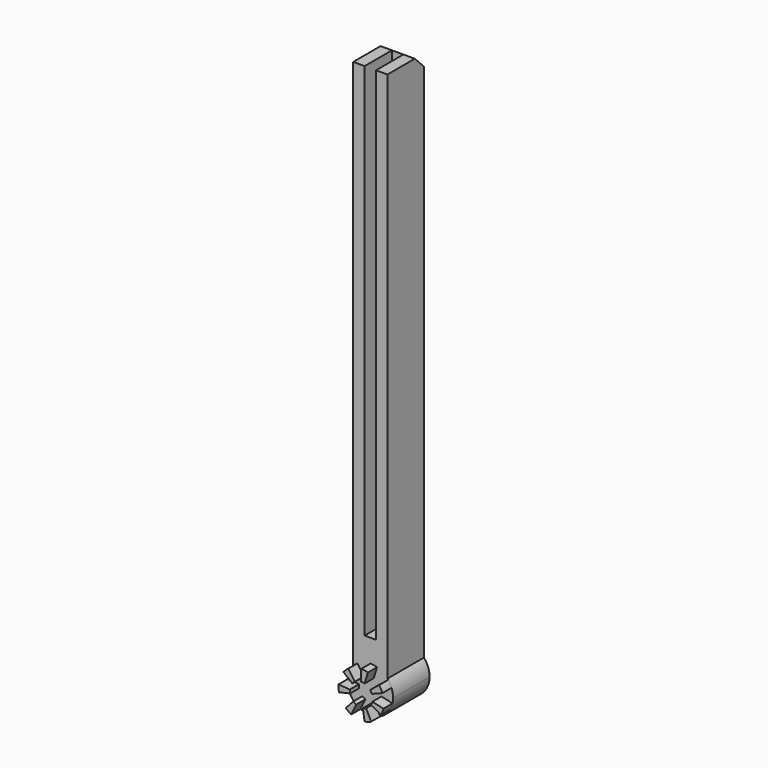
from build123d import *

# Parameters (mm, degrees)
F1_DEPTH = 12.7
F2_W     = 3.175
F2_H     = 9.525
F3_DEPTH = 139.7
F5_DEPTH = 3.175
F6_R     = 3.96875
F7_DEPTH = 3.175
F8_SIZE  = 3.17499


# Not quite as in the source:
# - a fillet or chamfer is up to 0.001 mm smaller than in the source, because OpenCascade refuses the exact size


with BuildPart() as f1:
    # F0 (on Front) → F1 (new body)
    with BuildSketch(Plane.XZ):
        with BuildLine():
            Line((0, 152.4), (0, 4.2001302063))
            ThreePointArc((0, 4.2001302063), (4.7625, 6.35), (9.525, 4.2001302063))
            Line((9.525, 4.2001302063), (9.525, 152.4))
            Line((9.525, 152.4), (0, 152.4))
        make_face()
        with BuildLine():
            Line((0, 4.2001302063), (0, 0))
            Line((0, 0), (9.525, 0))
            Line((9.525, 0), (9.525, 4.2001302063))
            ThreePointArc((9.525, 4.2001302063), (4.7625, 6.35), (0, 4.2001302063))
        make_face()
        with BuildLine():
            Line((9.525, 0), (0, 0))
            Line((0, 0), (0, 4.2001302063))
            ThreePointArc((0, 4.2001302063), (2.5174359697, -5.9398811015), (11.1125, 0))
            ThreePointArc((11.1125, 0), (10.7023811015, 2.2450640303), (9.525, 4.2001302063))
            Line((9.525, 4.2001302063), (9.525, 0))
        make_face()
    extrude(amount=F1_DEPTH)

    # F2 (on face) → F3 (cut)
    with BuildSketch(Plane.XY.offset(152.4)):
        with Locations((4.7625, -7.9375)):
            Rectangle(F2_W, F2_H)
    extrude(amount=-F3_DEPTH, mode=Mode.SUBTRACT)

    # F4 (on face) → F5 (join)
    with BuildSketch(Plane.XZ.offset(12.7)):
        with BuildLine():
            Line((5.2357091951, -3.1395378733), (5.7089183902, -6.2790757465))
            ThreePointArc((5.7089183902, -6.2790757465), (6.6341953575, -6.0678873167), (7.5176617434, -5.7211523112))
            Line((7.5176617434, -5.7211523112), (6.1400808717, -2.8605761556))
            ThreePointArc((6.1400808717, -2.8605761556), (5.6983476788, -3.0339436584), (5.2357091951, -3.1395378733))
        make_face()
        with BuildLine():
            Line((2.6029515576, -2.3274396931), (0.4434031152, -4.6548793861))
            ThreePointArc((0.4434031152, -4.6548793861), (1.1854176313, -5.2466162169), (2.0073382566, -5.7211523112))
            Line((2.0073382566, -5.7211523112), (3.3849191283, -2.8605761556))
            ThreePointArc((3.3849191283, -2.8605761556), (2.9739588156, -2.6233081085), (2.6029515576, -2.3274396931))
        make_face()
        with BuildLine():
            Line((1.5963779439, 0.2372680471), (-1.5697441121, 0.4745360943))
            ThreePointArc((-1.5697441121, 0.4745360943), (-1.5697441121, -0.4745360943), (-1.4282922424, -1.4130079306))
            Line((-1.4282922424, -1.4130079306), (1.6671038788, -0.7065039653))
            ThreePointArc((1.6671038788, -0.7065039653), (1.5963779439, -0.2372680471), (1.5963779439, 0.2372680471))
        make_face()
        with BuildLine():
            ThreePointArc((2.2801850432, 1.9795801209), (2.6029515576, 2.3274396931), (2.9739588156, 2.6233081085))
            Line((2.9739588156, 2.6233081085), (1.1854176313, 5.2466162169))
            ThreePointArc((1.1854176313, 5.2466162169), (0.5600076724, 4.760415763), (0, 4.2001302063))
            ThreePointArc((0, 4.2001302063), (-0.1025571138, 4.080896872), (-0.2021299137, 3.9591602418))
            Line((-0.2021299137, 3.9591602418), (2.2801850432, 1.9795801209))
        make_face()
        with BuildLine():
            Line((4.7625, 6.35), (4.7625, 3.175))
            ThreePointArc((4.7625, 3.175), (5.2357091951, 3.1395378733), (5.6983476788, 3.0339436584))
            Line((5.6983476788, 3.0339436584), (6.6341953575, 6.0678873167))
            ThreePointArc((6.6341953575, 6.0678873167), (5.7089183902, 6.2790757465), (4.7625, 6.35))
        make_face()
        with BuildLine():
            ThreePointArc((10.6735483039, 2.3199155047), (10.261761314, 3.175), (9.7271299137, 3.9591602418))
            Line((9.7271299137, 3.9591602418), (7.2448149568, 1.9795801209))
            ThreePointArc((7.2448149568, 1.9795801209), (7.512130657, 1.5875), (7.7180241519, 1.1599577524))
            Line((7.7180241519, 1.1599577524), (10.6735483039, 2.3199155047))
        make_face()
        with BuildLine():
            Line((7.512130657, -1.5875), (10.261761314, -3.175))
            ThreePointArc((10.261761314, -3.175), (10.6735483039, -2.3199155047), (10.9532922424, -1.4130079306))
            Line((10.9532922424, -1.4130079306), (7.8578961212, -0.7065039653))
            ThreePointArc((7.8578961212, -0.7065039653), (7.7180241519, -1.1599577524), (7.512130657, -1.5875))
        make_face()
    extrude(amount=F5_DEPTH)

    # F6 (on face) → F7 (cut)
    with BuildSketch(Plane(origin=(0, 0, 0), x_dir=(-1, 0, 0), z_dir=(0, 1, 0))):
        with Locations((-4.7625, 0)):
            Circle(F6_R)
    extrude(amount=-F7_DEPTH, mode=Mode.SUBTRACT)

    # F8 (size 3.175 in the source; OpenCascade refuses exactly that, so slightly less here)
    f8_edges = [f1.edges().sort_by_distance(p)[0] for p in [
        (4.7625, 0, 152.4),
    ]]
    chamfer(f8_edges, length=F8_SIZE)


solid = f1.part
